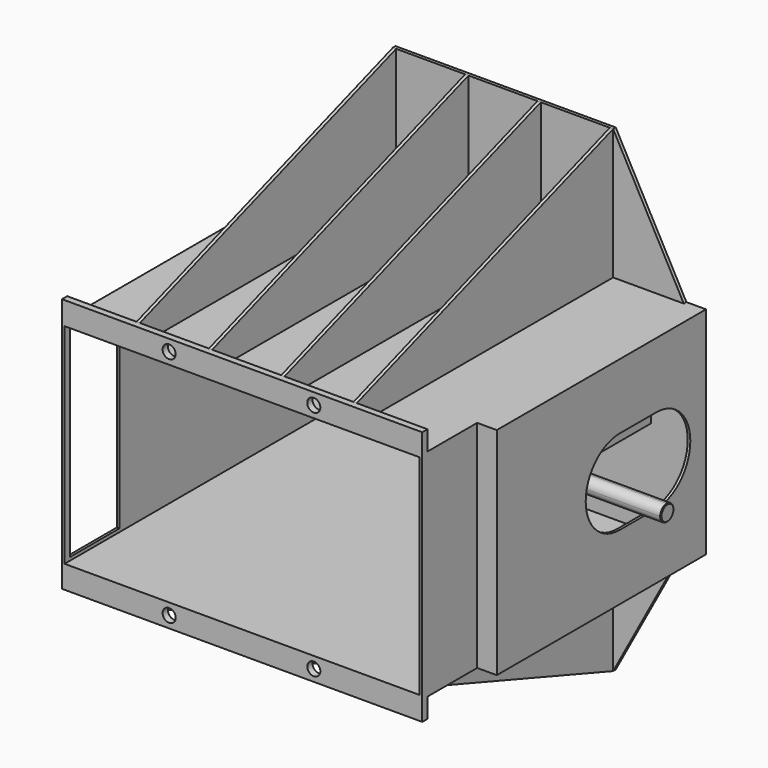
from build123d import *

# Parameters (mm, degrees)
F0_W      = 753
F0_H      = 730
F1_DEPTH  = 5
F2_W      = 551
F2_H      = 330
F2_W_2    = 543
F2_H_2    = 320
F3_DEPTH  = 500
F4_W      = 10
F4_H      = 30
F5_DEPTH  = 551
F6_W      = 5
F6_H      = 200
F7_DEPTH  = 490
F10_DEPTH = 546.401
F13_DEPTH = 5.001
F15_DEPTH = 30
F16_W     = 390
F16_H     = 320
F17_DEPTH = 30
F18_W     = 70
F18_H     = 130
F19_DEPTH = 5
F20_W     = 95
F20_H     = 310
F21_DEPTH = 5
F22_W     = 25
F22_H     = 25
F23_DEPTH = 200
F25_DEPTH = 175
F27_R     = 10
F28_DEPTH = 25


# Not quite as in the source:
# - a fillet or chamfer that OpenCascade refuses, or shapes differently, is made with other operations: its cross-section is extruded or revolved along the edge and cut away or added


with BuildPart() as f1:
    # F0 (on Front) → F1 (new body)
    with BuildSketch(Plane.XZ):
        Rectangle(F0_W, F0_H)
    extrude(amount=F1_DEPTH)

    # F2 (on face) → F3 (join)
    with BuildSketch(Plane.XZ.offset(5)):
        with Locations((-0.5, 0)):
            Rectangle(F2_W, F2_H)
        with Locations((-0.5, 0)):
            Rectangle(F2_W_2, F2_H_2, mode=Mode.SUBTRACT)
    extrude(amount=F3_DEPTH)

    # F4 (on face) → F5 (join, through all)
    with BuildSketch(Plane(origin=(-276, 0, 0), x_dir=(0, -1, 0), z_dir=(-1, 0, 0))):
        with Locations((500, 180)):
            Rectangle(F4_W, F4_H)
        with Locations((500, -180)):
            Rectangle(F4_W, F4_H)
    extrude(amount=-F5_DEPTH)

    # F6 (on face) → F7 (join, through all)
    with BuildSketch(Plane.XZ.offset(5)):
        with Locations((164.4, 265)):
            Rectangle(F6_W, F6_H)
        with Locations((53.8, 265)):
            Rectangle(F6_W, F6_H)
        with Locations((-56.8, 265)):
            Rectangle(F6_W, F6_H)
        with Locations((-167.4, 265)):
            Rectangle(F6_W, F6_H)
        with Locations((164.4, -265)):
            Rectangle(F6_W, F6_H)
        with Locations((53.8, -265)):
            Rectangle(F6_W, F6_H)
        with Locations((-56.8, -265)):
            Rectangle(F6_W, F6_H)
        with Locations((-167.4, -265)):
            Rectangle(F6_W, F6_H)
    extrude(amount=F7_DEPTH)

    # F8 (on face) + F9 (on face) → F10 (cut, through all)
    with BuildSketch(Plane(origin=(-169.9, 0, 0), x_dir=(0, -1, 0), z_dir=(-1, 0, 0))):
        Polygon((5, 365), (495, 195), (495, 365), align=None)
    with BuildSketch(Plane(origin=(-169.9, 0, 0), x_dir=(0, -1, 0), z_dir=(-1, 0, 0))):
        Polygon((495, -365), (495, -195), (5, -365), align=None)
    extrude(amount=-F10_DEPTH, mode=Mode.SUBTRACT)

    # F11 (on face) + F12 (on face) → F13 (cut, through all)
    with BuildSketch(Plane.XZ.offset(5)):
        Polygon((275, -165), (166.9, -365), (376.5, -365), (376.5, 365), (166.9, 365), (275, 165), align=None)
    with BuildSketch(Plane.XZ.offset(5)):
        Polygon((-376.5, -365), (-169.9, -365), (-276, -165), (-276, 165), (-169.9, 365), (-376.5, 365), align=None)
    extrude(amount=-F13_DEPTH, mode=Mode.SUBTRACT)

    # F14 (on face) → F15 (join)
    with BuildSketch(Plane.YZ.offset(275)):
        Polygon((-5, -165), (0, -165), (0, 165), (-5, 165), (-400, 165), (-400, -165), align=None)
    extrude(amount=F15_DEPTH)

    # F16 (on face) → F17 (cut)
    with BuildSketch(Plane(origin=(271, 0, 0), x_dir=(0, -1, 0), z_dir=(-1, 0, 0))):
        with Locations((200, 0)):
            Rectangle(F16_W, F16_H)
    extrude(amount=-F17_DEPTH, mode=Mode.SUBTRACT)

    # F18 (on face) → F19 (cut)
    with BuildSketch(Plane.YZ.offset(305)):
        with BuildLine():
            ThreePointArc((-165, 65), (-230, 0), (-165, -65))
            Line((-165, -65), (-165, 65))
        make_face()
        with Locations((-130, 0)):
            Rectangle(F18_W, F18_H)
        with BuildLine():
            Line((-95, 65), (-95, -65))
            ThreePointArc((-95, -65), (-30, 0), (-95, 65))
        make_face()
    extrude(amount=-F19_DEPTH, mode=Mode.SUBTRACT)

    # F20 (on face) → F21 (cut)
    with BuildSketch(Plane(origin=(-276, 0, 0), x_dir=(0, -1, 0), z_dir=(-1, 0, 0))):
        with Locations((447.5, 0)):
            Rectangle(F20_W, F20_H)
    extrude(amount=-F21_DEPTH, mode=Mode.SUBTRACT)

    # F22 (on face) → F23 (join)
    with BuildSketch(Plane.XZ.offset(5)):
        with Locations((212.5, 0)):
            Rectangle(F22_W, F22_H)
    extrude(amount=F23_DEPTH)

    # F24 (on face) → F25 (join)
    with BuildSketch(Plane.YZ.offset(225)):
        with BuildLine():
            ThreePointArc((-192.5, -12.5), (-183.6611652352, -8.8388347648), (-180, 0))
            ThreePointArc((-180, 0), (-183.6611652352, 8.8388347648), (-192.5, 12.5))
            ThreePointArc((-192.5, 12.5), (-201.3388347648, 8.8388347648), (-205, 0))
            ThreePointArc((-205, 0), (-201.3388347648, -8.8388347648), (-192.5, -12.5))
        make_face()
    extrude(amount=F25_DEPTH)

    # F26: chamfer of 1.1 on 1 edges, made by hand

    # F26_s1 → F26_t2 (revolve, cut)
    with BuildSketch(Plane.XZ.offset(192.5)):
        Polygon((398.9, 12.5), (400, 11.4), (400, 12.5), align=None)
    revolve(axis=Axis((400, -192.5, 0), (-1, 0, 0)), mode=Mode.SUBTRACT)

    # F27 (on face) → F28 (cut)
    with BuildSketch(Plane.XZ.offset(505)):
        with Locations((109.1, 177.5)):
            Circle(F27_R)
        with Locations((-112.1, 177.5)):
            Circle(F27_R)
        with Locations((-112.1, -177.5)):
            Circle(F27_R)
        with Locations((109.1, -177.5)):
            Circle(F27_R)
    extrude(amount=-F28_DEPTH, mode=Mode.SUBTRACT)


solid = f1.part
